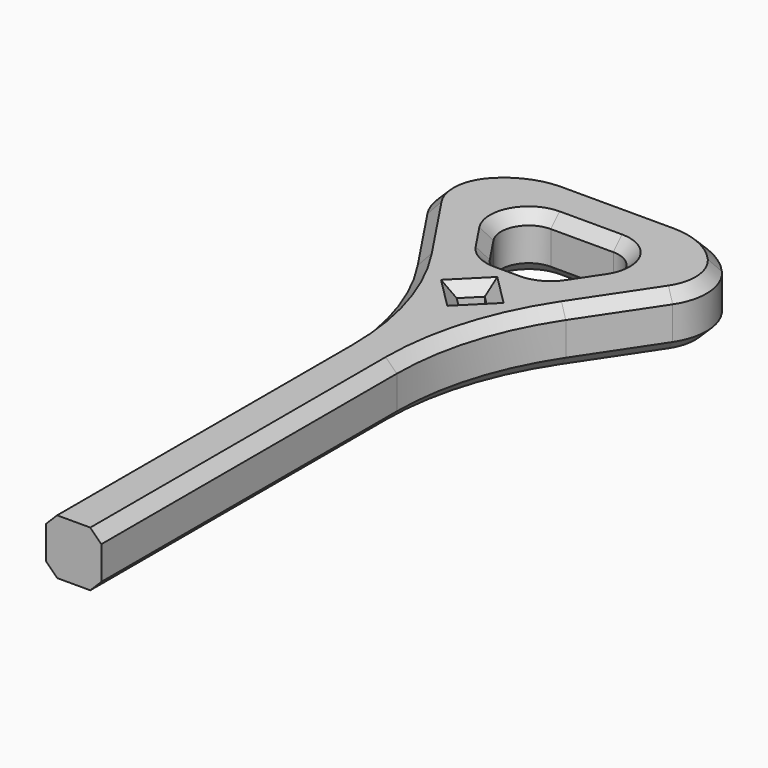
from build123d import *

# Parameters (mm, degrees)
F0_W        = 30
F0_H        = 10
F1_DEPTH    = 10
F2_R        = 5
F3_T1_DEPTH = 84.348882825
F4_R        = 10
F5_R        = 50
F6_SIZE     = 2
F8_DEPTH    = 10.001
F9_SIZE     = 2


# Not quite as in the source:
# - a fillet or chamfer that OpenCascade refuses, or shapes differently, is made with other operations: its cross-section is extruded or revolved along the edge and cut away or added


with BuildPart() as f1:
    # F0 (on Top) → F1 (new body)
    with BuildSketch(Plane.XY):
        Polygon((5, 50), (-5, 50), (-15, 65), (-15, 75), (-25, 75), (-25, 61.9722436227), (-5, 31.9722436227), (-5, -50), (5, -50), (5, 31.9722436227), (25, 61.9722436227), (25, 75), (15, 75), (15, 65), align=None)
        with Locations((0, 70)):
            Rectangle(F0_W, F0_H)
    extrude(amount=F1_DEPTH)

    # F2
    f2_edges = [f1.edges().sort_by_distance(p)[0] for p in [
        (15, 65, 5),
        (-15, 65, 5),
        (-5, 50, 5),
        (5, 50, 5),
    ]]
    fillet(f2_edges, radius=F2_R)

    # F3: fillet of radius 15 on 2 edges, made by hand

    # F3_s2 → F3_t1 (cut)
    with BuildSketch(Plane.XY.offset(-37.1744414125)):
        with BuildLine():
            ThreePointArc((-25, 61.9722436227), (-20.0149678844, 71.2823679771), (-10.130223435, 75))
            Line((-10.130223435, 75), (-25, 75))
            Line((-25, 75), (-25, 61.9722436227))
        make_face()
        with BuildLine():
            ThreePointArc((25, 61.9722436227), (20.0149678844, 71.2823679771), (10.130223435, 75))
            Line((10.130223435, 75), (25, 75))
            Line((25, 75), (25, 61.9722436227))
        make_face()
    extrude(amount=F3_T1_DEPTH, mode=Mode.SUBTRACT)

    # F4
    f4_edges = [f1.edges().sort_by_distance(p)[0] for p in [
        (-25, 61.972244, 5),
        (25, 61.972244, 5),
    ]]
    fillet(f4_edges, radius=F4_R)

    # F5
    f5_edges = [f1.edges().sort_by_distance(p)[0] for p in [
        (5, 31.972244, 5),
        (-5, 31.972244, 5),
    ]]
    fillet(f5_edges, radius=F5_R)

    # F6
    f6_edges = [f1.edges().sort_by_distance(p)[0] for p in [
        (0, 65, 10),
        (0, 75, 10),
        (0, 50, 0),
        (0, 75, 0),
    ]]
    chamfer(f6_edges, length=F6_SIZE)

    # F7 (on face) → F8 (cut, through all)
    with BuildSketch(Plane.XY.offset(10)):
        Polygon((0, 37.3431457505), (2.8284271247, 40.1715728753), (0, 43), (-2.8284271247, 40.1715728753), align=None)
    extrude(amount=-F8_DEPTH, mode=Mode.SUBTRACT)

    # F9
    f9_edges = [f1.edges().sort_by_distance(p)[0] for p in [
        (1.414214, 41.585786, 10),
        (-1.414214, 41.585786, 10),
        (1.414214, 38.757359, 10),
        (-1.414214, 38.757359, 10),
        (1.414214, 38.757359, 0),
        (1.414214, 41.585786, 0),
        (-1.414214, 41.585786, 0),
        (-1.414214, 38.757359, 0),
    ]]
    chamfer(f9_edges, length=F9_SIZE)


solid = f1.part
